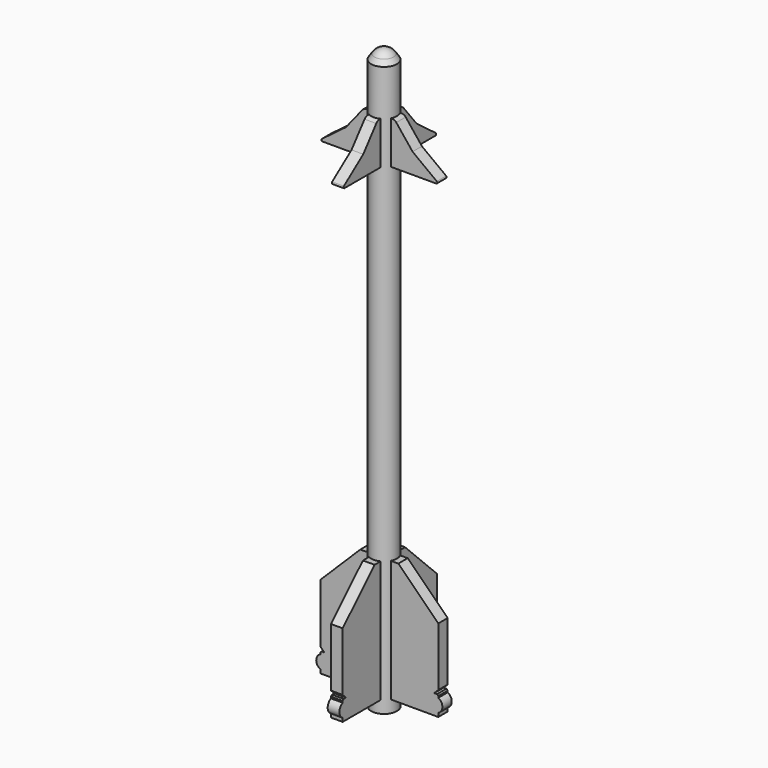
from build123d import *

# Parameters (mm, degrees)
F3_DEPTH = 0.2
F5_COUNT = 4


# Not quite as in the source:
# - a feature of the source that left no trace in its solid (it failed there, or was rolled back) is left out


with BuildPart() as f1:
    # F0 (on Front) → F1 (revolve)
    with BuildSketch(Plane.XZ):
        with BuildLine():
            Line((0, 19.7916666667), (0, 0))
            Line((0, 0), (0.4409722222, 0))
            Line((0.4409722222, 0), (0.4409722222, 19.4444444444))
            Line((0.4409722222, 19.4444444444), (0.3249042511, 19.6180555556))
            ThreePointArc((0.3249042511, 19.6180555556), (0.1841898411, 19.745542126), (0, 19.7916666667))
        make_face()
    revolve(axis=Axis((0, 0, 9.8958333333), (0, 0, 1)))

    # F2 (on Front) → F3 (join, symmetric)
    with BuildSketch(Plane.XZ):
        with BuildLine():
            Line((2.0138888889, 3.2291666667), (0.6493055556, 4.5833333333))
            Line((0.6493055556, 4.5833333333), (-0.6493055556, 4.5833333333))
            Line((-0.6493055556, 4.5833333333), (-2.0138888889, 3.2291666667))
            Line((-2.0138888889, 3.2291666667), (-2.0138888889, 1.2291666667))
            Line((-2.0138888889, 1.2291666667), (-1.875, 1.0902777778))
            Line((-1.875, 1.0902777778), (-1.9722222222, 1.0902777778))
            Line((-1.9722222222, 1.0902777778), (-2.0138888889, 1.0486111111))
            Line((-2.0138888889, 1.0486111111), (-2.0138888889, 0.9930555556))
            ThreePointArc((-2.0138888889, 0.9930555556), (-2.1527777778, 0.7673611111), (-2.0138888889, 0.5416666667))
            Line((-2.0138888889, 0.5416666667), (-2.0138888889, 0.4166666667))
            Line((-2.0138888889, 0.4166666667), (2.0138888889, 0.4166666667))
            Line((2.0138888889, 0.4166666667), (2.0138888889, 0.5416666667))
            ThreePointArc((2.0138888889, 0.5416666667), (2.1527777778, 0.7673611111), (2.0138888889, 0.9930555556))
            Line((2.0138888889, 0.9930555556), (2.0138888889, 1.0486111111))
            Line((2.0138888889, 1.0486111111), (1.9722222222, 1.0902777778))
            Line((1.9722222222, 1.0902777778), (1.875, 1.0902777778))
            Line((1.875, 1.0902777778), (2.0138888889, 1.2291666667))
            Line((2.0138888889, 1.2291666667), (2.0138888889, 3.2291666667))
        make_face()
        with BuildLine():
            Line((0.4409722222, 17.8819444444), (-0.4409722222, 17.8819444444))
            ThreePointArc((-0.4409722222, 17.8819444444), (-0.5180541376, 17.8643461976), (-0.5798611111, 17.8150388148))
            Line((-0.5798611111, 17.8150388148), (-1.1354166667, 17.1180555556))
            Line((-1.1354166667, 17.1180555556), (-1.9632069856, 16.4955808322))
            ThreePointArc((-1.9632069856, 16.4955808322), (-1.9771060186, 16.4509380855), (-1.9391666667, 16.4236111111))
            Line((-1.9391666667, 16.4236111111), (1.9391666667, 16.4236111111))
            ThreePointArc((1.9391666667, 16.4236111111), (1.9771060186, 16.4509380855), (1.9632069856, 16.4955808322))
            Line((1.9632069856, 16.4955808322), (1.1354166667, 17.1180555556))
            Line((1.1354166667, 17.1180555556), (0.5798611111, 17.8150388148))
            ThreePointArc((0.5798611111, 17.8150388148), (0.5180541376, 17.8643461976), (0.4409722222, 17.8819444444))
        make_face()
    extrude(amount=F3_DEPTH, both=True)

    # F5: F1 ×4 about axis
    f5_axis = Axis((0, 0, 0), (0, 0, 1))


with BuildPart() as f1_1:
    add(f1.part)
    for i in range(1, F5_COUNT):
        add(f1.part.rotate(f5_axis, i * 360 / F5_COUNT))


solid = f1_1.part
